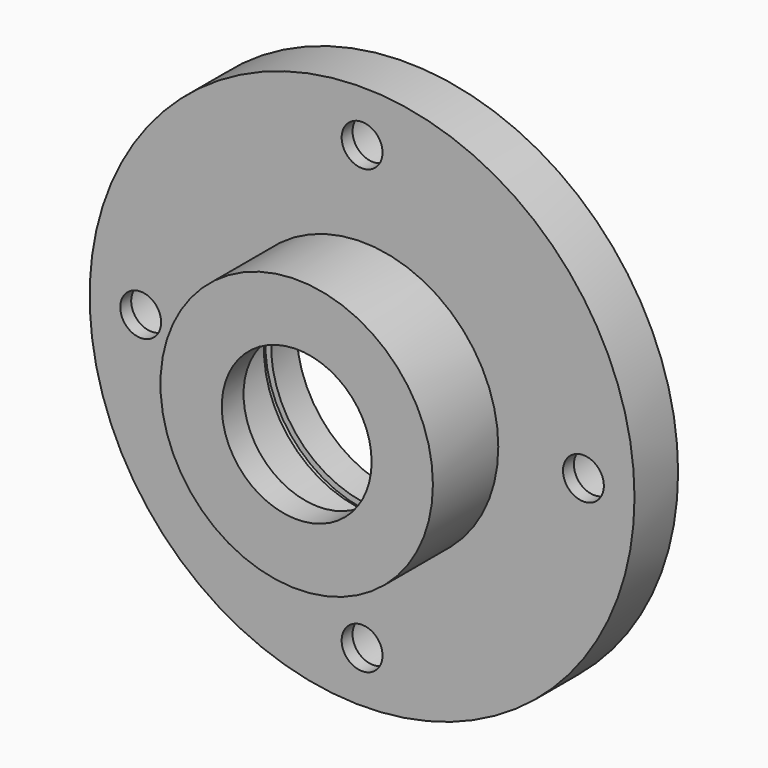
from build123d import *

# Parameters (mm, degrees)
F3_D            = 6
F3_COPIES_COUNT = 4
F4_R            = 5
F4_R_2          = 3
F5_DEPTH        = 6
F5_COPIES_COUNT = 4


# Not quite as in the source:
# - a pattern or mirror of a feature is missing from the dataset's text; its kind, count and spacing are read off the source's solid


with BuildPart() as f1:
    # F0 (on Top) → F1 (revolve)
    with BuildSketch(Plane.XY):
        Polygon((47.481939, -5.127659), (47.481939, 2.872341), (23.481939, 2.872341), (23.481939, -1.827659), (24.331939, -1.827659), (24.331939, -3.127659), (23.481939, -3.127659), (23.481939, -13.127659), (18.481939, -13.127659), (18.481939, -17.127659), (27.481939, -17.127659), (27.481939, -5.127659), align=None)
    revolve(axis=Axis((7.481939, -6.8666535, 0), (0, -1, 0)))

    # F3 (through all)
    with Locations(Plane(origin=(0, 2.872341, 0), x_dir=(-1, 0, 0), z_dir=(0, 1, 0))):
        with Locations((-7.481939, 32.5)):
            f3 = Hole(F3_D / 2)

    # F3_copies: F3 ×4 about axis
    f3_copies_axis = Axis((7.481939, 0, 0), (0, 1, 0))
    for i in range(1, F3_COPIES_COUNT):
        add(f3.rotate(f3_copies_axis, i * 360 / F3_COPIES_COUNT), mode=Mode.SUBTRACT)

    # F4 (on face) → F5 (cut)
    with BuildSketch(Plane(origin=(0, 2.872341, 0), x_dir=(-1, 0, 0), z_dir=(0, 1, 0))):
        with Locations((-7.481939, 32.5)):
            Circle(F4_R)
        with Locations((-7.481939, 32.5)):
            Circle(F4_R_2, mode=Mode.SUBTRACT)
    f5 = extrude(amount=-F5_DEPTH, mode=Mode.SUBTRACT)

    # F5_copies: F5 ×4 about axis
    f5_copies_axis = Axis((7.481939, 0, 0), (0, 1, 0))
    for i in range(1, F5_COPIES_COUNT):
        add(f5.rotate(f5_copies_axis, i * 360 / F5_COPIES_COUNT), mode=Mode.SUBTRACT)


solid = f1.part
